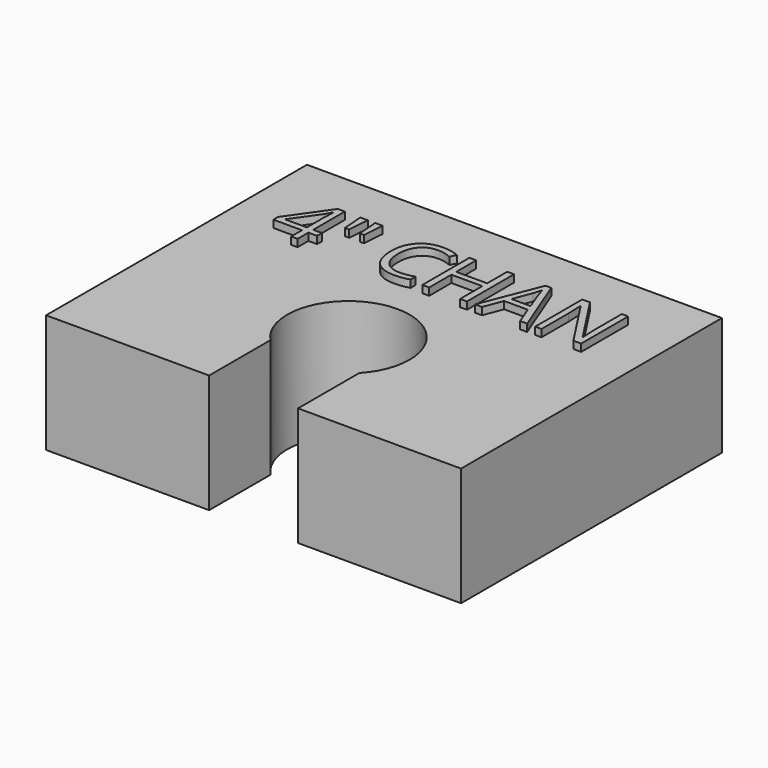
from build123d import *

# Parameters (mm, degrees)
F0_W         = 88.9
F0_H         = 69.85
F1_DEPTH     = 25.4
F3_DEPTH     = 25.4
F4_TEXT_SIZE = 17.6388888889
F5_DEPTH     = 1.5748


# Not quite as in the source:
# - Text() gives the source's letters only with a copy of the font that has no kerning and outlines rounded to 1/6400 em; it was checked with that copy


with BuildPart() as f1:
    # F0 (on Top) → F1 (new body)
    with BuildSketch(Plane.XY):
        with Locations((-8.6369048804, 14.2642892237)):
            Rectangle(F0_W, F0_H)
    extrude(amount=F1_DEPTH)

    # F2 (on face) → F3 (cut)
    with BuildSketch(Plane.XY.offset(25.4)):
        with BuildLine():
            Line((0.8880951196, -20.6607107763), (0.8880951196, -4.2497324008))
            ThreePointArc((0.8880951196, -4.2497324008), (-8.6369048804, 17.8361642237), (-18.1619048804, -4.2497324008))
            Line((-18.1619048804, -4.2497324008), (-18.1619048804, -20.6607107763))
            Line((-18.1619048804, -20.6607107763), (0.8880951196, -20.6607107763))
        make_face()
    extrude(amount=-F3_DEPTH, mode=Mode.SUBTRACT)

    # F4 (on face) → F5 (join)
    with BuildSketch(Plane.XY.offset(25.4)):
        with Locations((-43.5150515818, 24.8893319713)):
            Text('4" CHAN', F4_TEXT_SIZE, font='Open Sans', text_align=(TextAlign.LEFT, TextAlign.BOTTOM))
    extrude(amount=F5_DEPTH)


solid = f1.part
